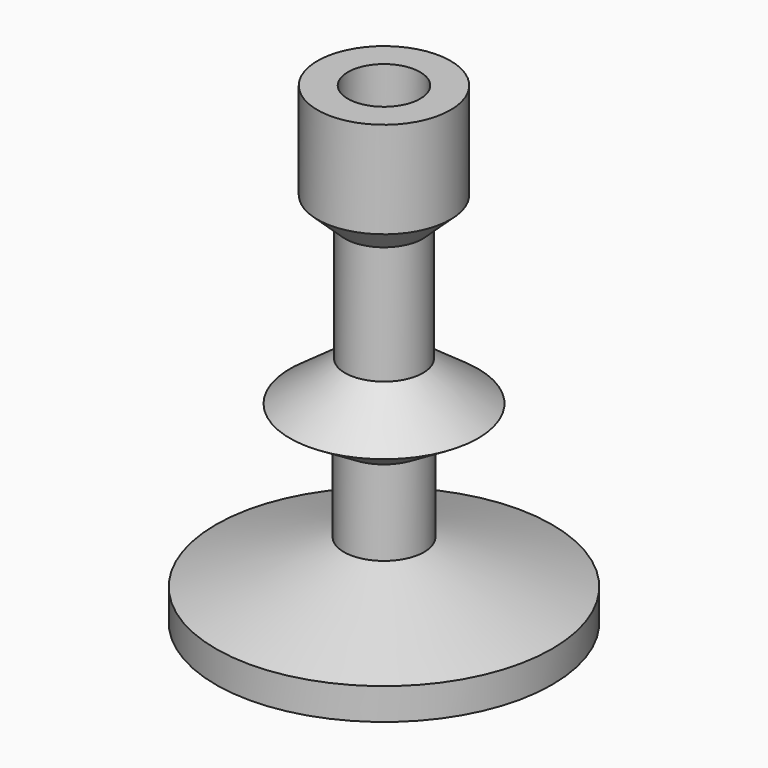
from build123d import *


# Not quite as in the source:
# - the program builds the solid bodies; features that only make, move or delete a surface that nothing else refers to are left out


with BuildPart() as f1:
    # F0 (on Front) → F1 (revolve)
    with BuildSketch(Plane.XZ):
        Polygon((9.4487518072, 56.2424510717), (0, 56.2424510717), (0, -56.0924559832), (43.9441055059, -56.0924559832), (43.9441055059, -47.8435605764), (10.498598218, -36.4450961351), (10.498598218, -14.248073101), (24.5967060328, -5.6992173195), (10.1986378431, 4.6493858099), (10.1986378431, 35.5452299118), (17.3976719379, 42.2943234444), (17.3976719379, 67.4909353256), (9.4487518072, 67.4909353256), align=None)
    revolve(axis=Axis((0, 0, 0.0749975443), (0, 0, 1)))


solid = f1.part
